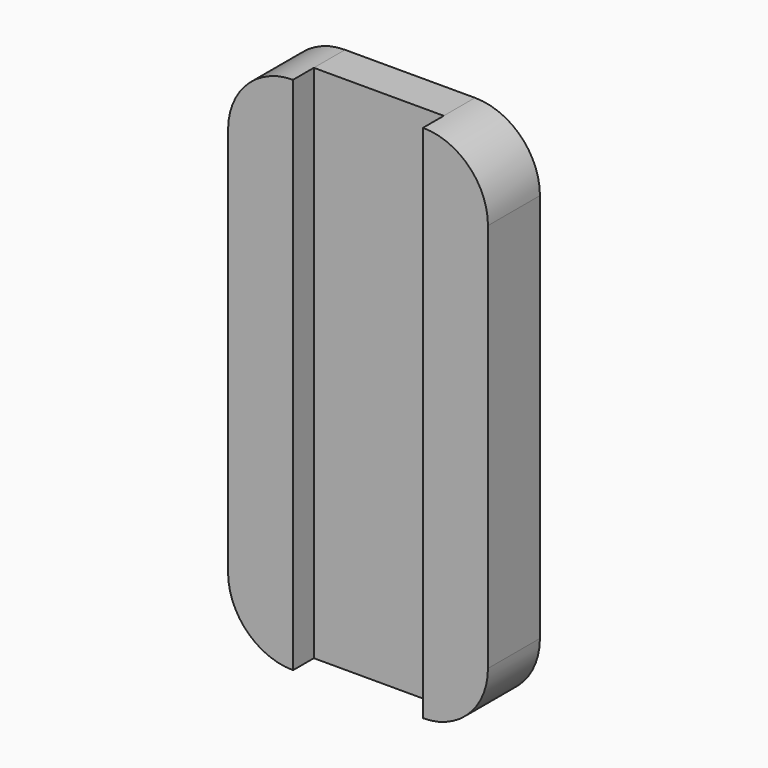
from build123d import *

# Parameters (mm, degrees)
F0_W     = 20
F0_H     = 40
F1_DEPTH = 5
F2_W     = 5
F2_H     = 2
F3_DEPTH = 40.001
F4_R     = 4.99999


# Not quite as in the source:
# - a fillet or chamfer is up to 0.001 mm smaller than in the source, because OpenCascade refuses the exact size


with BuildPart() as f1:
    # F0 (on Front) → F1 (new body)
    with BuildSketch(Plane.XZ):
        Rectangle(F0_W, F0_H)
    extrude(amount=F1_DEPTH)

    # F2 (on face) → F3 (cut, through all)
    with BuildSketch(Plane(origin=(0, 0, -20), x_dir=(1, 0, 0), z_dir=(0, 0, -1))):
        with Locations((-2.5, 4)):
            Rectangle(F2_W, F2_H)
        with Locations((2.5, 4)):
            Rectangle(F2_W, F2_H)
    extrude(amount=-F3_DEPTH, mode=Mode.SUBTRACT)

    # F4 (radius 5 in the source; OpenCascade refuses exactly that, so slightly less here)
    f4_edges = [f1.edges().sort_by_distance(p)[0] for p in [
        (-10, -2.5, -20),
        (10, -2.5, -20),
        (-10, -2.5, 20),
        (10, -2.5, 20),
    ]]
    fillet(f4_edges, radius=F4_R)


solid = f1.part
